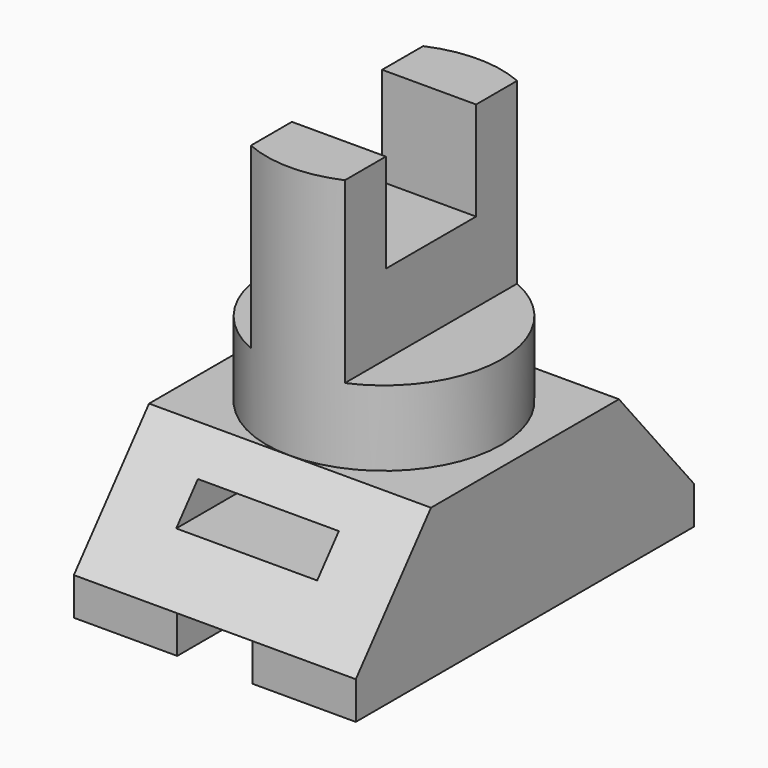
from build123d import *

# Parameters (mm, degrees)
F1_DEPTH  = 30
F2_R      = 25
F3_DEPTH  = 54
F4_W      = 50
F4_H      = 24
F5_DEPTH  = 21
F6_W      = 25
F6_H      = 50
F7_DEPTH  = 38
F8_W      = 30
F8_H      = 9
F11_W     = 16
F11_H     = 8
F12_DEPTH = 90.001


# Not quite as in the source:
# - a pattern or mirror of a feature is missing from the dataset's text; its kind, count and spacing are read off the source's solid


with BuildPart() as f1:
    # F0 (on Right) → F1 (new body, symmetric)
    with BuildSketch(Plane.YZ):
        Polygon((-45, 0), (0, 0), (45, 0), (45, 8), (25, 32), (0, 32), (-25, 32), (-45, 8), align=None)
    extrude(amount=F1_DEPTH, both=True)

    # F2 (on face) → F3 (join)
    with BuildSketch(Plane.XY.offset(32)):
        Circle(F2_R)
    extrude(amount=F3_DEPTH)

    # F4 (on face) → F5 (cut)
    with BuildSketch(Plane.XY.offset(86)):
        Rectangle(F4_W, F4_H)
    extrude(amount=-F5_DEPTH, mode=Mode.SUBTRACT)

    # F6 (on face) → F7 (cut)
    with BuildSketch(Plane.XY.offset(86)):
        with Locations((22.5, 0)):
            Rectangle(F6_W, F6_H)
    f7 = extrude(amount=-F7_DEPTH, mode=Mode.SUBTRACT)

    # F7_copies: F7 across plane
    add(f7.mirror(Plane(origin=(0, 0, 0), x_dir=(0, 0, -1), z_dir=(-1, 0, 0))), mode=Mode.SUBTRACT)

    # F10: sweep along a path in F9
    with BuildLine(Plane.YZ.offset(30)) as f10_path:
        Line((-35, 20), (51.1633306742, 20))
    # F8 (on face) → F10 (sweep, cut)
    with BuildSketch(Plane(origin=(0, -30.4918032787, 25.4098360656), x_dir=(1, 0, 0), z_dir=(0, -0.7682212796, 0.6401843997))):
        with Locations((0, -4.9215290445)):
            Rectangle(F8_W, F8_H)
    sweep(path=f10_path.line, mode=Mode.SUBTRACT)

    # F11 (on face) → F12 (cut, through all)
    with BuildSketch(Plane.XZ.offset(45)):
        with Locations((0, 4)):
            Rectangle(F11_W, F11_H)
    extrude(amount=-F12_DEPTH, mode=Mode.SUBTRACT)


solid = f1.part
